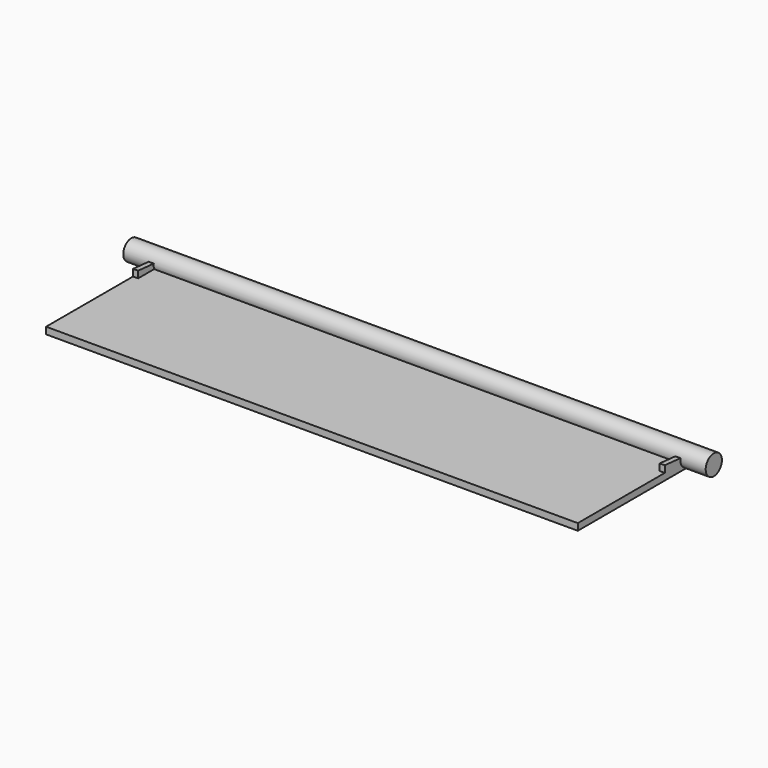
from build123d import *

# Parameters (mm, degrees)
F0_W     = 137.8
F0_H     = 2.4
F3_DEPTH = 62.9
F4_START = -61.7
F4_DEPTH = 1.2


with BuildPart() as f1:
    # F0 (on Top) → F1 (revolve)
    with BuildSketch(Plane.XY):
        with Locations((0, 1.2)):
            Rectangle(F0_W, F0_H)
    revolve(axis=Axis((-37.6928597689, 0, 0), (1, 0, 0)))

    # F2 (on Right) → F3 (join, symmetric)
    with BuildSketch(Plane.YZ):
        Polygon((-32.72, -2.4), (0, -2.4), (0, -0.8), (-7, -0.8), (-32.72, -0.8), align=None)
    extrude(amount=F3_DEPTH, both=True)

    # F2 (on Right) → F4 (join)
    with BuildSketch(Plane.YZ.offset(F4_START)):
        Polygon((-7, -0.8), (0, -0.8), (0, 0.1875793553), (-7, 0.8), align=None)
    extrude(amount=-F4_DEPTH)

    # F5: F1 across plane


with BuildPart() as f1_1:
    add(f1.part)
    add(f1.part.mirror(Plane.YZ))


solid = f1_1.part
